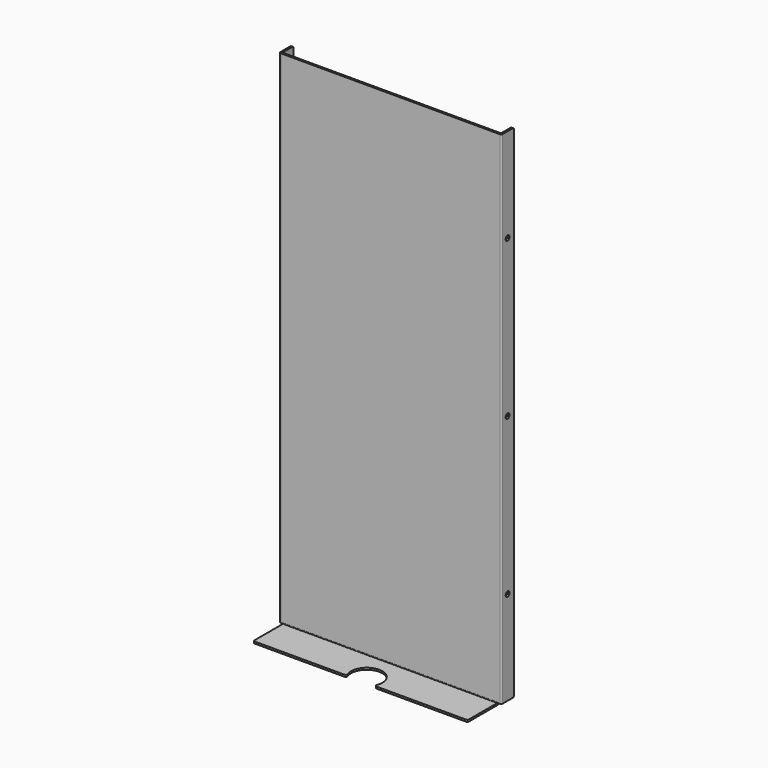
from build123d import *

# Parameters (mm, degrees)
F0_W     = 180.086
F0_H     = 406.4
F1_DEPTH = 12.7
F2_T     = -1.524
F3_R     = 2
F4_DEPTH = 180.087
F5_W     = 173.736
F5_H     = 1.524
F6_DEPTH = 31.75
F8_DEPTH = 25.4
F9_R     = 1.27
F10_R    = 0.508


with BuildPart() as f1:
    # F0 (on Front) → F1 (new body)
    with BuildSketch(Plane.XZ):
        with Locations((0, 203.2)):
            Rectangle(F0_W, F0_H)
    extrude(amount=-F1_DEPTH)

    # F2
    f2_openings = [f1.faces().sort_by_distance(p)[0] for p in [
        (0, 6.35, 406.4),
        (0, 6.35, 0),
        (0, 12.7, 203.2),
    ]]
    offset(amount=F2_T, openings=f2_openings)

    # F3 (on face) → F4 (cut, through all)
    with BuildSketch(Plane.YZ.offset(90.043)):
        with Locations((6.35, 76.2)):
            Circle(F3_R)
        with Locations((6.35, 330.2)):
            Circle(F3_R)
        with Locations((6.35, 203.2)):
            Circle(F3_R)
    extrude(amount=-F4_DEPTH, mode=Mode.SUBTRACT)

    # F5 (on face) → F6 (join)
    with BuildSketch(Plane(origin=(0, 1.524, 0), x_dir=(-1, 0, 0), z_dir=(0, 1, 0))):
        with Locations((0, -0.762)):
            Rectangle(F5_W, F5_H)
    extrude(amount=-F6_DEPTH)

    # F7 (on face) → F8 (cut)
    with BuildSketch(Plane(origin=(0, 0, -1.524), x_dir=(1, 0, 0), z_dir=(0, 0, -1))):
        with BuildLine():
            ThreePointArc((-10.9985226281, 30.226), (-3.2870018728, 11.6087420061), (12.7, 23.876))
            ThreePointArc((12.7, 23.876), (12.2672579939, 27.1630018728), (10.9985226281, 30.226))
            Line((10.9985226281, 30.226), (-10.9985226281, 30.226))
        make_face()
    extrude(amount=-F8_DEPTH, mode=Mode.SUBTRACT)

    # F9
    f9_edges = [f1.edges().sort_by_distance(p)[0] for p in [
        (90.043, 0, 203.2),
        (0, 1.524, -1.524),
        (-90.043, 0, 203.2),
        (-10.998523, -30.226, -0.762),
        (10.998523, -30.226, -0.762),
        (-86.868, -30.226, -0.762),
        (86.868, -30.226, -0.762),
        (-89.281, 12.7, 0),
        (89.281, 12.7, 0),
        (89.281, 12.7, 406.4),
        (-89.281, 12.7, 406.4),
    ]]
    fillet(f9_edges, radius=F9_R)

    # F10
    f10_edges = [f1.edges().sort_by_distance(p)[0] for p in [
        (-88.519, 1.524, 203.2),
        (88.519, 1.524, 203.2),
        (0, 0, 0),
    ]]
    fillet(f10_edges, radius=F10_R)


solid = f1.part
